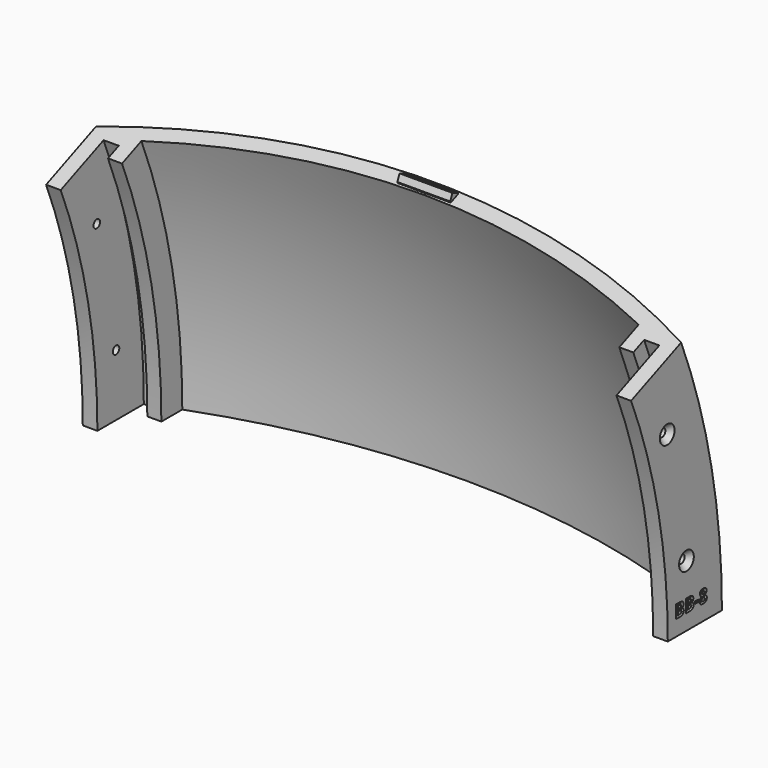
from build123d import *

# Parameters (mm, degrees)
F0_W         = 18.0700589621
F0_H         = 3.4022678406
F1_ANGLE     = 22.5
F3_TEXT_SIZE = 6.2362746879
F4_DEPTH     = 1
F5_ANGLE     = 23
F6_ANGLE     = 0.5
F2_R         = 1.4
F7_DEPTH     = 139.36235
F8_SIZE      = 1.75
F9_T1_DEPTH  = 26.8722322136
F9_T3_DEPTH  = 26.7853820393
F10_T1_DEPTH = 26.8722322136
F10_T3_DEPTH = 26.7853820393


# Not quite as in the source:
# - a fillet or chamfer that OpenCascade refuses, or shapes differently, is made with other operations: its cross-section is extruded or revolved along the edge and cut away or added
# - a feature names something its author has since deleted; it is built from what else it names
# - Text() gives the source's letters only with a copy of the font that has no kerning and outlines rounded to 1/6400 em; it was checked with that copy


with BuildPart() as f1:
    # F0 (on Top) → F1 (revolve)
    with BuildSketch(Plane.XY):
        with BuildLine():
            Line((-95, 206), (-95, 225.8317958127))
            ThreePointArc((-95, 225.8317958127), (-90.0216753203, 227.8620152033), (-85, 229.7825058615))
            ThreePointArc((-85, 229.7825058615), (0, 245), (85, 229.7825058615))
            ThreePointArc((85, 229.7825058615), (90.0216753203, 227.8620152033), (95, 225.8317958127))
            Line((95, 225.8317958127), (95, 206))
            Line((95, 206), (100, 206))
            Line((100, 206), (100, 229.1287847478))
            ThreePointArc((100, 229.1287847478), (0, 250), (-100, 229.1287847478))
            Line((-100, 229.1287847478), (-100, 206))
            Line((-100, 206), (-95, 206))
        make_face()
        with Locations((0, 247.3350245834)):
            Rectangle(F0_W, F0_H, mode=Mode.SUBTRACT)
        with BuildLine():
            ThreePointArc((-85, 229.7825058615), (-90.0216753203, 227.8620152033), (-95, 225.8317958127))
            Line((-95, 225.8317958127), (-94, 225.8317958127))
            Line((-94, 225.8317958127), (-89.8, 225.8317958127))
            Line((-89.8, 225.8317958127), (-89.8, 220.8317958127))
            Line((-89.8, 220.8317958127), (-85, 220.8317958127))
            Line((-85, 220.8317958127), (-85, 229.7825058615))
        make_face()
        with BuildLine():
            ThreePointArc((95, 225.8317958127), (90.0216753203, 227.8620152033), (85, 229.7825058615))
            Line((85, 229.7825058615), (85, 220.8317958127))
            Line((85, 220.8317958127), (89.8, 220.8317958127))
            Line((89.8, 220.8317958127), (89.8, 225.8317958127))
            Line((89.8, 225.8317958127), (94, 225.8317958127))
            Line((94, 225.8317958127), (95, 225.8317958127))
        make_face()
        with Locations((0, 247.3350245834)):
            Rectangle(F0_W, F0_H)
    revolve(axis=Axis((0, 0, 0), (1, 0, 0)), revolution_arc=F1_ANGLE)

    # F3 (on face) → F4 (cut)
    with BuildSketch(Plane.YZ.offset(100)):
        with Locations((208.9602351189, 5.3157305811)):
            Text('BB-8', F3_TEXT_SIZE, font='Open Sans', font_style=FontStyle.BOLD, text_align=(TextAlign.LEFT, TextAlign.BOTTOM))
    extrude(amount=-F4_DEPTH, mode=Mode.SUBTRACT)

    # F0 (on Top) → F5 (revolve)
    with BuildSketch(Plane.XY):
        with Locations((0, 247.3350245834)):
            Rectangle(F0_W, F0_H)
    revolve(axis=Axis((0, 0, 0), (1, 0, 0)), revolution_arc=F5_ANGLE)

    # F2 (on Right) → F7 (cut, symmetric)
    with BuildSketch(Plane.YZ):
        with Locations((205.7421721824, 62.4112056097)):
            Circle(F2_R)
        with Locations((213.9647162345, 21.0736851709)):
            Circle(F2_R)
    extrude(amount=F7_DEPTH, both=True, mode=Mode.SUBTRACT)

    # F8
    f8_edges = [f1.edges().sort_by_distance(p)[0] for p in [
        (100, 212.564716, 21.073685),
        (100, 204.342172, 62.411206),
        (-100, 212.564716, 21.073685),
        (-100, 204.342172, 62.411206),
    ]]
    chamfer(f8_edges, length=F8_SIZE)

    # F9: chamfer of 1.7 on 2 edges, made by hand

    # F9_s2 → F9_t1 (cut)
    with BuildSketch(Plane.YZ.offset(-13.4361161068)):
        with BuildLine():
            Line((229.9023861575, 95.728266888), (227.6687564527, 96.6396535519))
            Line((227.6687564527, 96.6396535519), (229.2389925878, 97.3061792468))
            ThreePointArc((229.2389925878, 97.3061792468), (229.5813608449, 96.4956319989), (229.9023861575, 95.728266888))
        make_face()
    extrude(amount=F9_T1_DEPTH, mode=Mode.SUBTRACT)

    # F9_s4 → F9_t3 (cut)
    with BuildSketch(Plane.YZ.offset(-13.3926910196)):
        with BuildLine():
            Line((226.761524936, 94.4204376761), (227.6666688451, 96.6387674151))
            Line((227.6666688451, 96.6387674151), (226.1071885278, 95.976807294))
            ThreePointArc((226.1071885278, 95.976807294), (226.4450115033, 95.1770193247), (226.761524936, 94.4204376761))
        make_face()
    extrude(amount=F9_T3_DEPTH, mode=Mode.SUBTRACT)


with BuildPart() as f6:
    # F0 (on Top) → F6 (revolve)
    with BuildSketch(Plane.XY):
        with Locations((0, 247.3350245834)):
            Rectangle(F0_W, F0_H)
    revolve(axis=Axis((0, 0, 0), (1, 0, 0)), revolution_arc=F6_ANGLE)

    # F10: chamfer of 1.7 on 2 edges, made by hand

    # F10_s2 → F10_t1 (cut)
    with BuildSketch(Plane.YZ.offset(-13.4361161068)):
        with BuildLine():
            Line((249.0840677411, 0.4137239879), (247.2725616551, 2.206165013))
            Line((247.2725616551, 2.206165013), (247.2722649529, 2.2401637184))
            ThreePointArc((247.2722649529, 2.2401637184), (248.1495326302, 2.1995694583), (249.0263792677, 2.2072215829))
            Line((249.0263792677, 2.2072215829), (249.0606746753, 2.1735195798))
            ThreePointArc((249.0606746753, 2.1735195798), (249.0667995338, 1.2935327826), (249.1180676827, 0.413787002))
            Line((249.1180676827, 0.413787002), (249.0840677411, 0.4137239879))
        make_face()
    extrude(amount=F10_T1_DEPTH, mode=Mode.SUBTRACT)

    # F10_s4 → F10_t3 (cut)
    with BuildSketch(Plane.YZ.offset(-13.3926910196)):
        with BuildLine():
            Line((245.5856405942, 0.4068941827), (247.3664590255, 2.2066539393))
            Line((247.3664590255, 2.2066539393), (247.3661623233, 2.2406526447))
            ThreePointArc((247.3661623233, 2.2406526447), (246.495410727, 2.1851341551), (245.624240975, 2.1775315719))
            Line((245.624240975, 2.1775315719), (245.5905389718, 2.1432361643))
            ThreePointArc((245.5905389718, 2.1432361643), (245.5965802629, 1.2751693454), (245.5516406526, 0.4068311708))
            Line((245.5516406526, 0.4068311708), (245.5856405942, 0.4068941827))
        make_face()
    extrude(amount=F10_T3_DEPTH, mode=Mode.SUBTRACT)


with BuildPart() as f1_1:
    add(f1.part)

    # F11: cut F6
    add(f6.part, mode=Mode.SUBTRACT)


solid = f1_1.part
